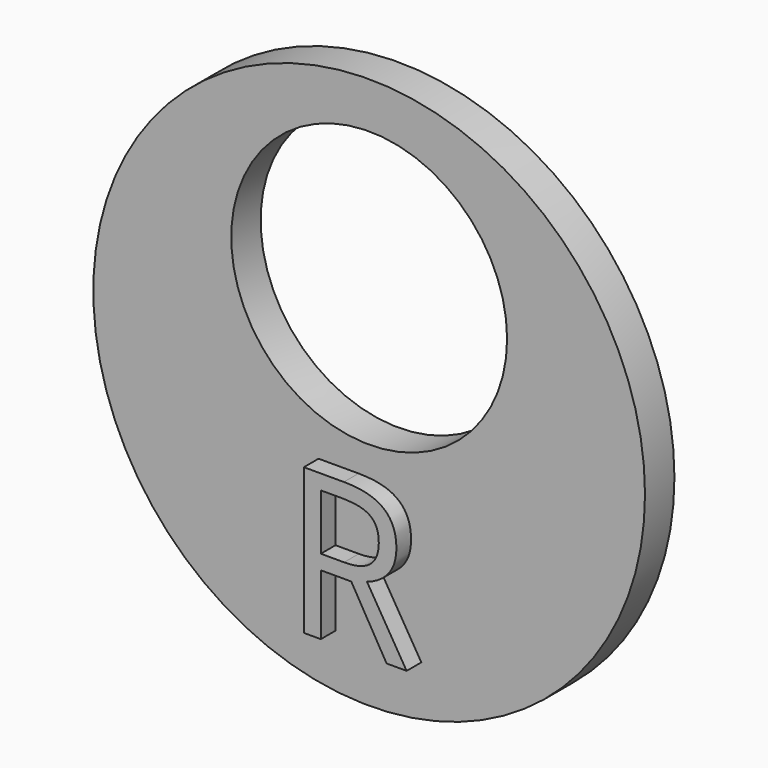
from build123d import *

# Parameters (mm, degrees)
F0_R         = 15
F0_R_2       = 7.5
F1_DEPTH     = 2
F2_TEXT_SIZE = 11.1111111111
F3_DEPTH     = 1


# Not quite as in the source:
# - Text() gives the source's letters only with a copy of the font that has no kerning and outlines rounded to 1/6400 em; it was checked with that copy


with BuildPart() as f1:
    # F0 (on Front) → F1 (new body)
    with BuildSketch(Plane.XZ):
        Circle(F0_R)
        with Locations((0, 5)):
            Circle(F0_R_2, mode=Mode.SUBTRACT)
    extrude(amount=F1_DEPTH)

    # F2 (on face) → F3 (join)
    with BuildSketch(Plane.XZ.offset(2)):
        with Locations((-3.840904932, -11.9975052006)):
            Text('R', F2_TEXT_SIZE, font='Open Sans', text_align=(TextAlign.LEFT, TextAlign.BOTTOM))
    extrude(amount=F3_DEPTH)


solid = f1.part
